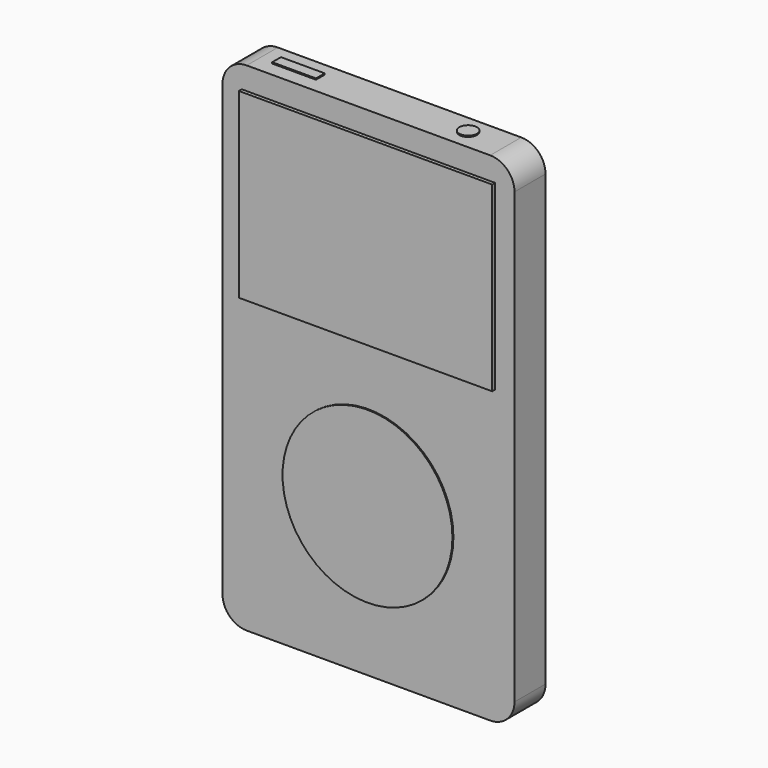
from build123d import *

# Parameters (mm, degrees)
F0_W      = 61.1160316085
F0_H      = 104.14
F1_DEPTH  = 8.128
F2_R      = 5.08
F4_W      = 9.1636627913
F4_H      = 2.2909147665
F4_R      = 1.8469945904
F5_DEPTH  = 0.254
F6_W      = 23.6879978329
F6_H      = 2.015999984
F7_DEPTH  = 0.254
F3_W      = 53.0287652906
F3_H      = 38.1
F8_DEPTH  = 0.762
F3_R      = 7.62
F9_DEPTH  = 0.254
F3_R_2    = 17.78
F10_DEPTH = 0.254


# Not quite as in the source:
# - the program builds the solid bodies; features that only make, move or delete a surface that nothing else refers to are left out


with BuildPart() as f1:
    # F0 (on Front) → F1 (new body)
    with BuildSketch(Plane.XZ):
        with Locations((-19.607455004, -3.8571991026)):
            Rectangle(F0_W, F0_H)
    extrude(amount=F1_DEPTH)

    # F2
    f2_edges = [f1.edges().sort_by_distance(p)[0] for p in [
        (10.950561, -4.064, 48.212801),
        (-50.165471, -4.064, 48.212801),
        (10.950561, -4.064, -55.927199),
        (-50.165471, -4.064, -55.927199),
    ]]
    fillet(f2_edges, radius=F2_R)

    # F4 (on face) → F5 (join)
    with BuildSketch(Plane.XY.offset(48.2128008974)):
        with Locations((-37.6597046852, -3.8777994923)):
            Rectangle(F4_W, F4_H)
        with Locations((-2.1505255718, -3.8777994923)):
            Circle(F4_R)
    extrude(amount=F5_DEPTH)

    # F6 (on face) → F7 (join)
    with BuildSketch(Plane(origin=(0, 0, -55.9271991026), x_dir=(1, 0, 0), z_dir=(0, 0, -1))):
        with Locations((-19.78199929, 4.4100000523)):
            Rectangle(F6_W, F6_H)
    extrude(amount=F7_DEPTH)

    # F3 (on face) → F8 (join)
    with BuildSketch(Plane.XZ.offset(8.128)):
        with Locations((-19.607455004, 24.4255777958)):
            Rectangle(F3_W, F3_H)
    extrude(amount=F8_DEPTH)

    # F3 (on face) → F9 (join)
    with BuildSketch(Plane.XZ.offset(8.128)):
        with Locations((-19.607455004, -24.6234625244)):
            Circle(F3_R)
    extrude(amount=F9_DEPTH)

    # F3 (on face) → F10 (join)
    with BuildSketch(Plane.XZ.offset(8.128)):
        with Locations((-19.607455004, -24.6234625244)):
            Circle(F3_R_2)
        with Locations((-19.607455004, -24.6234625244)):
            Circle(F3_R, mode=Mode.SUBTRACT)
    extrude(amount=F10_DEPTH)


solid = f1.part
